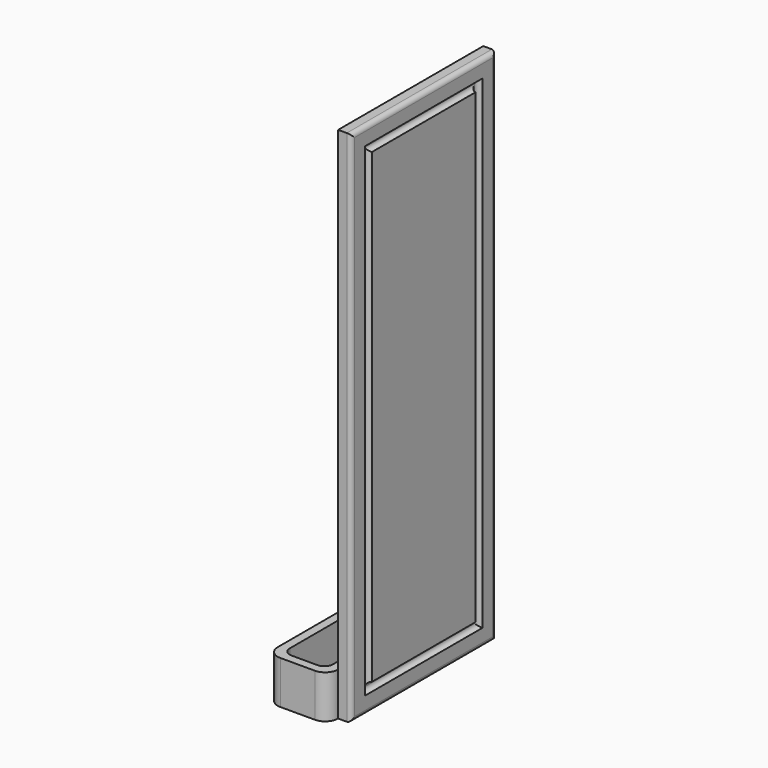
from build123d import *

# Parameters (mm, degrees)
F0_W     = 70
F0_H     = 240
F0_W_2   = 50
F0_H_2   = 220
F1_DEPTH = 50
F2_R     = 15
F3_R     = 10
F4_W     = 210
F4_H     = 50
F4_H_2   = 550
F5_DEPTH = 15
F6_W     = 170
F6_H     = 560
F6_W_2   = 150
F6_H_2   = 540
F7_DEPTH = 5
F8_R     = 4.99999
F9_R     = 5


# Not quite as in the source:
# - a fillet or chamfer is up to 0.001 mm smaller than in the source, because OpenCascade refuses the exact size


with BuildPart() as f1:
    # F0 (on Top) → F1 (new body)
    with BuildSketch(Plane.XY):
        with Locations((-35, 120)):
            Rectangle(F0_W, F0_H)
        with Locations((-35, 120)):
            Rectangle(F0_W_2, F0_H_2, mode=Mode.SUBTRACT)
    extrude(amount=F1_DEPTH)

    # F2
    f2_edges = [f1.edges().sort_by_distance(p)[0] for p in [
        (-70, 0, 25),
        (0, 0, 25),
        (-70, 240, 25),
        (0, 240, 25),
    ]]
    fillet(f2_edges, radius=F2_R)

    # F3
    f3_edges = [f1.edges().sort_by_distance(p)[0] for p in [
        (-10, 10, 25),
        (-60, 10, 25),
        (-10, 230, 25),
        (-60, 230, 25),
    ]]
    fillet(f3_edges, radius=F3_R)


with BuildPart() as f5:
    # F4 (on face) → F5 (new body)
    with BuildSketch(Plane.YZ):
        with Locations((120, 25)):
            Rectangle(F4_W, F4_H)
        with Locations((120, 325)):
            Rectangle(F4_W, F4_H_2)
    extrude(amount=F5_DEPTH)

    # F6 (on face) → F7 (cut)
    with BuildSketch(Plane.YZ.offset(15)):
        with Locations((120, 300)):
            Rectangle(F6_W, F6_H)
        with Locations((120, 300)):
            Rectangle(F6_W_2, F6_H_2, mode=Mode.SUBTRACT)
    extrude(amount=-F7_DEPTH, mode=Mode.SUBTRACT)

    # F8 (radius 5 in the source; OpenCascade refuses exactly that, so slightly less here)
    f8_edges = [f5.edges().sort_by_distance(p)[0] for p in [
        (10, 120, 20),
        (10, 120, 30),
        (10, 35, 300),
        (10, 120, 580),
        (10, 195, 300),
        (10, 45, 300),
        (10, 120, 570),
        (10, 205, 300),
    ]]
    fillet(f8_edges, radius=F8_R)

    # F9
    f9_edges = [f5.edges().sort_by_distance(p)[0] for p in [
        (15, 120, 0),
        (15, 225, 300),
        (15, 15, 300),
        (15, 120, 600),
    ]]
    fillet(f9_edges, radius=F9_R)


solid = Compound([f1.part, f5.part])
